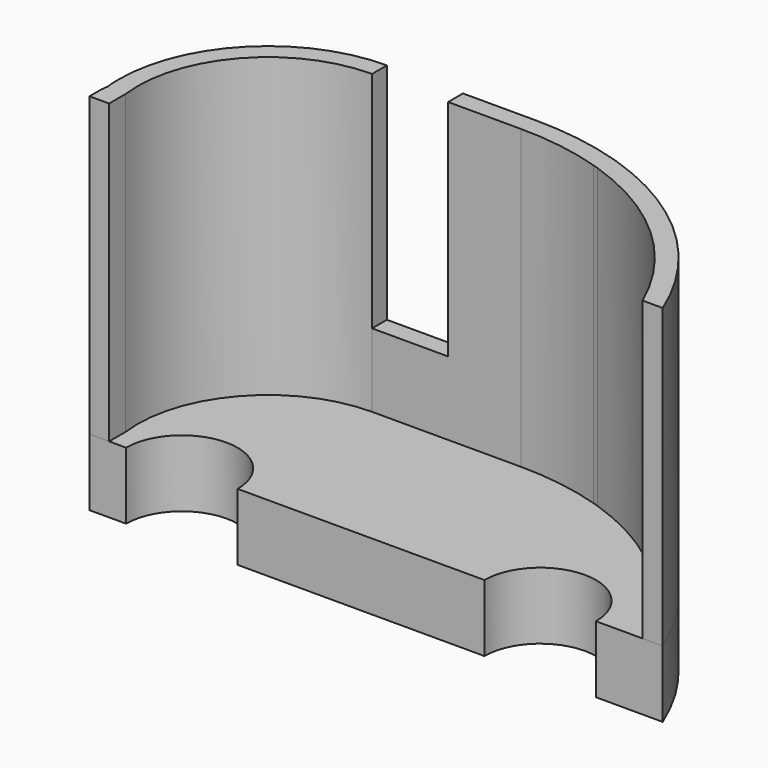
from build123d import *

# Parameters (mm, degrees)
F1_DEPTH = 22.86
F3_DEPTH = 101.6
F4_W     = 25.9639685869
F4_H     = 76.5026504314
F5_DEPTH = 25.4


# Not quite as in the source:
# - ends of sketch curves that miss each other by under 0.0002 mm in the source are joined


with BuildPart() as f1:
    # F0 (on Top) → F1 (new body)
    with BuildSketch(Plane.XY):
        with BuildLine():
            Line((54.1491188765, 51.4247583449), (3.3491188765, 51.4247583449))
            ThreePointArc((3.3491188765, 51.4247583449), (-32.5719056078, 36.5457828292), (-47.4508811235, 0.6247583449))
            Line((-47.4508811235, 0.6247583449), (-47.4508811235, -12.0752416551))
            Line((-47.4508811235, -12.0752416551), (-34.9568908542, -12.0752416551))
            ThreePointArc((-34.9568908542, -12.0752416551), (-15.9068908542, 6.9747583449), (3.1431091458, -12.0752416551))
            Line((3.1431091458, -12.0752416551), (87.4382129431, -12.0752416551))
            ThreePointArc((87.4382129431, -12.0752416551), (106.4882129431, 6.9747583449), (125.5382129431, -12.0752416551))
            Line((125.5382129431, -12.0752416551), (148.3348396626, -12.0752416551))
            ThreePointArc((148.3348396626, -12.0752416551), (110.945245505, 34.0670280199), (54.1491188765, 51.4247583449))
        make_face()
    extrude(amount=F1_DEPTH)


with BuildPart() as f3:
    # F2 (on face) → F3 (new body)
    with BuildSketch(Plane.XY.offset(22.86)):
        with BuildLine():
            Line((15.9320533276, 51.4247583449), (3.3491188765, 51.4247583449))
            ThreePointArc((3.3491188765, 51.4247583449), (-32.5719056078, 36.5457828292), (-47.4508811235, 0.6247583449))
            ThreePointArc((-47.4508811235, 0.6247583449), (-47.3782321455, -2.091094798), (-47.1604930017, -4.7991800686))
            ThreePointArc((-47.1604930017, -4.7991800686), (-47.3280960303, -5.9197039916), (-47.4508811235, -7.0460203141))
            Line((-47.4508811235, -7.0460203141), (-47.4508811235, -12.0752416551))
            Line((-47.4508811235, -12.0752416551), (-40.7406055237, -12.0752416551))
            Line((-40.7406055237, -12.0752416551), (-40.7406055237, -5.0231332932))
            ThreePointArc((-40.7406055237, -5.0231332932), (-30.0189141756, 29.9910119001), (3.3491188765, 45.0747580933))
            Line((3.3491188765, 45.0747580933), (54.1491188765, 45.0747583449))
            ThreePointArc((54.1491188765, 45.0747583449), (68.3996721284, 44.0026988236), (82.3294388374, 40.8106490516))
            Line((82.3294388374, 40.8106490516), (84.3304985233, 40.1665928591))
            ThreePointArc((84.3304985233, 40.1665928591), (118.4348676457, 20.1092178361), (141.4471872445, -12.0752416551))
            Line((141.4471872445, -12.0752416551), (148.3348396626, -12.0752416551))
            ThreePointArc((148.3348396626, -12.0752416551), (123.7178725829, 23.8703423302), (86.3088204644, 46.2006557144))
            Line((86.3088204644, 46.2006557144), (84.242132955, 46.8658347181))
            ThreePointArc((84.242132955, 46.8658347181), (69.3673093156, 50.2785620546), (54.1491188765, 51.4247583449))
            Line((54.1491188765, 51.4247583449), (36.9653739035, 51.4247583449))
            Line((36.9653739035, 51.4247583449), (15.9320533276, 51.4247583449))
        make_face()
    extrude(amount=F3_DEPTH)

    # F4 (on face) → F5 (cut)
    with BuildSketch(Plane(origin=(0, 51.4247583449, 0), x_dir=(-1, 0, 0), z_dir=(0, 1, 0))):
        with Locations((-16.3311031699, 86.2086747843)):
            Rectangle(F4_W, F4_H)
    extrude(amount=-F5_DEPTH, mode=Mode.SUBTRACT)


solid = Compound([f1.part, f3.part])
